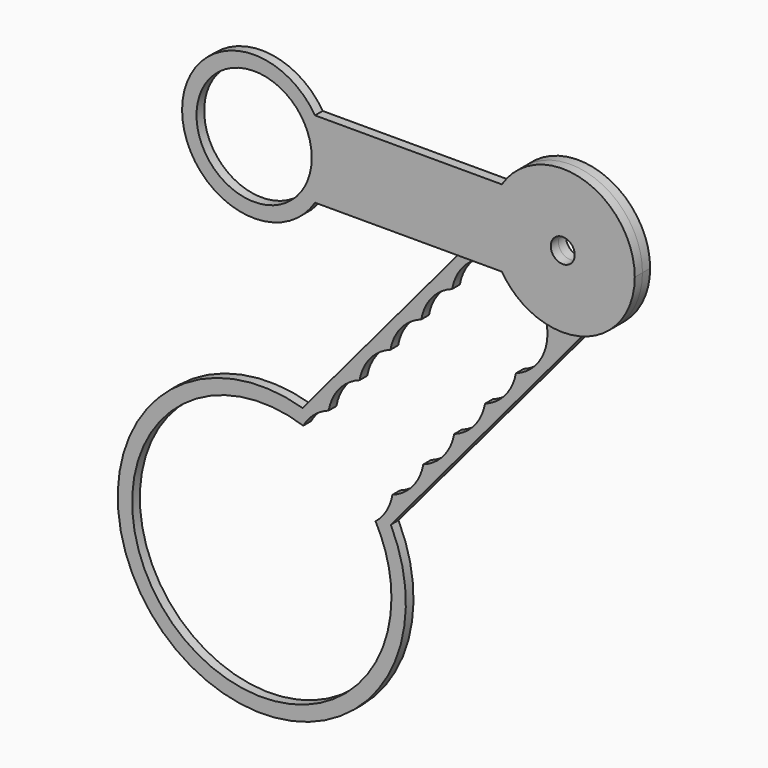
from build123d import *

# Parameters (mm, degrees)
F0_R     = 15.24
F0_R_2   = 3.175
F1_DEPTH = 2.54
F2_DEPTH = 2.54


with BuildPart() as f1:
    # F0 (on Front) → F1 (new body)
    with BuildSketch(Plane.XZ):
        with BuildLine():
            ThreePointArc((-65.5195329538, -10.16), (-63.3326111745, -5.287787783), (-62.5840264302, 0))
            ThreePointArc((-62.5840264302, 0), (-63.3326111745, 5.287787783), (-65.5195329538, 10.16))
            ThreePointArc((-65.5195329538, 10.16), (-100.6840264302, 0), (-65.5195329538, -10.16))
        make_face()
        with Locations((-81.6340264302, 0)):
            Circle(F0_R, mode=Mode.SUBTRACT)
        with BuildLine():
            ThreePointArc((-65.5195329538, 10.16), (-63.3326111745, 5.287787783), (-62.5840264302, 0))
            ThreePointArc((-62.5840264302, 0), (-63.3326111745, -5.287787783), (-65.5195329538, -10.16))
            Line((-65.5195329538, -10.16), (-28.4196593422, -10.16))
            Line((-28.4196593422, -10.16), (-19.0215796919, 1.0401951868))
            ThreePointArc((-19.0215796919, 1.0401951868), (-18.1501685771, 5.7856616408), (-16.1144934764, 10.16))
            Line((-16.1144934764, 10.16), (-65.5195329538, 10.16))
        make_face()
        with BuildLine():
            ThreePointArc((19.05, 0), (5.287787783, 18.3014152557), (-16.1144934764, 10.16))
            ThreePointArc((-16.1144934764, 10.16), (-18.1501685771, 5.7856616408), (-19.0215796919, 1.0401951868))
            ThreePointArc((-19.0215796919, 1.0401951868), (-18.4728068477, -4.6538056648), (-16.2583471742, -9.9281744125))
            ThreePointArc((-16.2583471742, -9.9281744125), (-10.6124234359, -12.6473937559), (-6.954110776, -17.7353557426))
            ThreePointArc((-6.954110776, -17.7353557426), (-1.3753346542, -19.0002882765), (4.3274549344, -18.5519711565))
            ThreePointArc((4.3274549344, -18.5519711565), (14.9221398683, -11.8419695047), (19.05, 0))
        make_face()
        Circle(F0_R_2, mode=Mode.SUBTRACT)
        with BuildLine():
            ThreePointArc((-16.2583471742, -9.9281744125), (-19.2670095389, -9.6856602103), (-22.2479261978, -10.16))
            Line((-22.2479261978, -10.16), (-16.1144934764, -10.16))
            ThreePointArc((-16.1144934764, -10.16), (-16.1868353523, -10.0443447411), (-16.2583471742, -9.9281744125))
        make_face()
        with BuildLine():
            Line((-19.0215796919, 1.0401951868), (-28.4196593422, -10.16))
            Line((-28.4196593422, -10.16), (-22.2479261978, -10.16))
            ThreePointArc((-22.2479261978, -10.16), (-19.2670095389, -9.6856602103), (-16.2583471742, -9.9281744125))
            ThreePointArc((-16.2583471742, -9.9281744125), (-18.4728068477, -4.6538056648), (-19.0215796919, 1.0401951868))
        make_face()
        with BuildLine():
            ThreePointArc((-6.954110776, -17.7353557426), (-10.6124234359, -12.6473937559), (-16.2583471742, -9.9281744125))
            ThreePointArc((-16.2583471742, -9.9281744125), (-16.1868353523, -10.0443447411), (-16.1144934764, -10.16))
            ThreePointArc((-16.1144934764, -10.16), (-12.1402895021, -14.6804588077), (-6.954110776, -17.7353557426))
        make_face()
    extrude(amount=F1_DEPTH)


with BuildPart() as f2:
    # F0 (on Front) → F2 (new body)
    with BuildSketch(Plane.XZ):
        with BuildLine():
            Line((-47.513862793, -80.334047803), (4.3274549344, -18.5519711565))
            ThreePointArc((4.3274549344, -18.5519711565), (-1.3753346542, -19.0002882765), (-6.954110776, -17.7353557426))
            ThreePointArc((-6.954110776, -17.7353557426), (-6.2973288868, -20.014568078), (-6.0758260789, -22.3761581835))
            ThreePointArc((-6.0758260789, -22.3761581835), (-8.3725951165, -29.6605789252), (-14.4321702587, -34.3102544675))
            ThreePointArc((-14.4321702587, -34.3102544675), (-17.2104642944, -40.2683252541), (-22.5955729017, -44.0390188951))
            ThreePointArc((-22.5955729017, -44.0390188951), (-25.3738669374, -49.9970896817), (-30.7589755447, -53.7677833227))
            ThreePointArc((-30.7589755447, -53.7677833227), (-33.5372695804, -59.7258541094), (-38.9223781878, -63.4965477503))
            ThreePointArc((-38.9223781878, -63.4965477503), (-41.7006722234, -69.454618537), (-47.0857808308, -73.2253121779))
            ThreePointArc((-47.0857808308, -73.2253121779), (-47.7541230349, -75.6172400855), (-48.8751976268, -77.8333610605))
            ThreePointArc((-48.8751976268, -77.8333610605), (-48.1711624462, -79.0709833859), (-47.513862793, -80.334047803))
        make_face()
        with BuildLine():
            ThreePointArc((-68.1638084144, -61.6482948628), (-69.5048829018, -61.1698664199), (-70.8628974193, -60.7418814597))
            ThreePointArc((-70.8628974193, -60.7418814597), (-112.1462372262, -120.1046333926), (-43.5340264302, -97.2876442761))
            ThreePointArc((-43.5340264302, -97.2876442761), (-44.542327665, -88.580412643), (-47.513862793, -80.334047803))
            ThreePointArc((-47.513862793, -80.334047803), (-48.1711624462, -79.0709833859), (-48.8751976268, -77.8333610605))
            ThreePointArc((-48.8751976268, -77.8333610605), (-50.0896781123, -79.44493893), (-51.5440882931, -80.8438088687))
            ThreePointArc((-51.5440882931, -80.8438088687), (-48.4106304665, -88.8017700937), (-47.3440264302, -97.2876442761))
            ThreePointArc((-47.3440264302, -97.2876442761), (-109.4901704698, -117.2836273539), (-70.6650727554, -64.7993978587))
            ThreePointArc((-70.6650727554, -64.7993978587), (-69.5400104718, -63.124172221), (-68.1638084144, -61.6482948628))
        make_face()
        with BuildLine():
            Line((-22.2479261978, -10.16), (-28.4196593422, -10.16))
            Line((-28.4196593422, -10.16), (-70.8628974193, -60.7418814597))
            ThreePointArc((-70.8628974193, -60.7418814597), (-69.5048829018, -61.1698664199), (-68.1638084144, -61.6482948628))
            ThreePointArc((-68.1638084144, -61.6482948628), (-66.1760278564, -60.1594265442), (-63.9364951143, -59.0858840376))
            ThreePointArc((-63.9364951143, -59.0858840376), (-61.1582010786, -53.1278132509), (-55.7730924713, -49.35711961))
            ThreePointArc((-55.7730924713, -49.35711961), (-52.9947984356, -43.3990488233), (-47.6096898282, -39.6283551824))
            ThreePointArc((-47.6096898282, -39.6283551824), (-44.8313957926, -33.6702843957), (-39.4462871852, -29.8995907547))
            ThreePointArc((-39.4462871852, -29.8995907547), (-36.6679931496, -23.9415199681), (-31.2828845422, -20.1708263271))
            ThreePointArc((-31.2828845422, -20.1708263271), (-28.2038448627, -13.8671945678), (-22.2479261978, -10.16))
        make_face()
        with BuildLine():
            Line((-19.0215796919, 1.0401951868), (-28.4196593422, -10.16))
            Line((-28.4196593422, -10.16), (-22.2479261978, -10.16))
            ThreePointArc((-22.2479261978, -10.16), (-19.2670095389, -9.6856602103), (-16.2583471742, -9.9281744125))
            ThreePointArc((-16.2583471742, -9.9281744125), (-18.4728068477, -4.6538056648), (-19.0215796919, 1.0401951868))
        make_face()
        with BuildLine():
            ThreePointArc((19.05, 0), (5.287787783, 18.3014152557), (-16.1144934764, 10.16))
            ThreePointArc((-16.1144934764, 10.16), (-18.1501685771, 5.7856616408), (-19.0215796919, 1.0401951868))
            ThreePointArc((-19.0215796919, 1.0401951868), (-18.4728068477, -4.6538056648), (-16.2583471742, -9.9281744125))
            ThreePointArc((-16.2583471742, -9.9281744125), (-10.6124234359, -12.6473937559), (-6.954110776, -17.7353557426))
            ThreePointArc((-6.954110776, -17.7353557426), (-1.3753346542, -19.0002882765), (4.3274549344, -18.5519711565))
            ThreePointArc((4.3274549344, -18.5519711565), (14.9221398683, -11.8419695047), (19.05, 0))
        make_face()
        Circle(F0_R_2, mode=Mode.SUBTRACT)
    extrude(amount=-F2_DEPTH)


solid = Compound([f1.part, f2.part])
